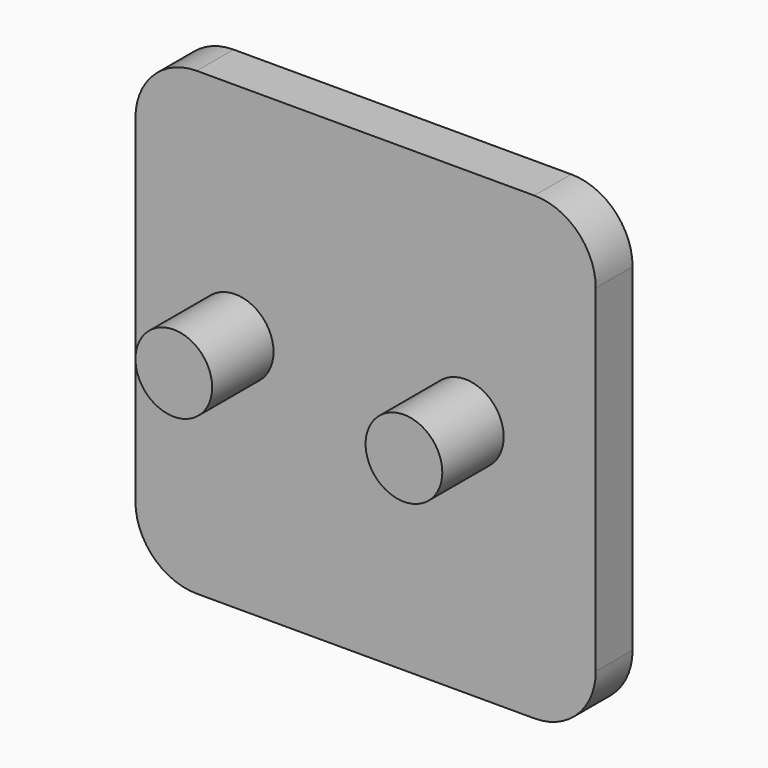
from build123d import *

# Parameters (mm, degrees)
F1_W           = 38.1
F1_H           = 38.1
F2_DEPTH       = 3.81
F3_R           = 3.175
F4_DEPTH       = 6.35
F5_R           = 5.08
F9_DEPTH       = 0.3175
F8_TEXT_SIZE   = 4.9309210024
F8_TEXT_SIZE_2 = 5.0353533071
F8_TEXT_SIZE_3 = 3.7948212897
F8_TEXT_SIZE_4 = 3.4233063666
F8_TEXT_SIZE_5 = 4.286538913
F8_TEXT_SIZE_6 = 3.7378385767
F8_TEXT_SIZE_7 = 4.2485771701
F8_TEXT_SIZE_8 = 4.0491771263
F10_DEPTH      = 0.3175
F11_W          = 23.3954964206
F11_H          = 0.4370380193
F12_DEPTH      = 0.3175


# Not quite as in the source:
# - Text() gives the source's letters only with a copy of the font that has no kerning and outlines rounded to 1/6400 em; it was checked with that copy


with BuildPart() as f2:
    # F1 (on offset) → F2 (new body)
    with BuildSketch(Plane.XZ.offset(25.4)):
        with Locations((-21.425308247, 18.5530144557)):
            Rectangle(F1_W, F1_H)
    extrude(amount=F2_DEPTH)

    # F3 (on face) → F4 (join)
    with BuildSketch(Plane.XZ.offset(29.21)):
        with Locations((-32.220308247, 19.1880144557)):
            Circle(F3_R)
        with Locations((-13.170308247, 19.1880144557)):
            Circle(F3_R)
    extrude(amount=F4_DEPTH)

    # F5
    f5_edges = [f2.edges().sort_by_distance(p)[0] for p in [
        (-40.475308, -27.305, 37.603014),
        (-2.375308, -27.305, 37.603014),
        (-40.475308, -27.305, -0.496986),
        (-2.375308, -27.305, -0.496986),
    ]]
    fillet(f5_edges, radius=F5_R)

    # F7 (on face) → F9 (cut)
    with BuildSketch(Plane(origin=(0, -25.4, 0), x_dir=(-1, 0, 0), z_dir=(0, 1, 0))):
        Polygon((12.6290200278, 34.7187258303), (3.9102202281, 34.7187258303), (6.485377904, 30.033910647), (6.8833935075, 5.9753647074), (6.922697669, 3.5995759973), (7.0077003911, 3.6009822506), (9.9715990946, 3.3956870902), (19.0850868821, 3.3956870902), (21.8502487987, 1.3529333519), (24.1223294288, 3.4225911368), (33.3103425801, 3.4225911368), (36.4377573133, 3.7207957357), (36.4377573133, 6.6668614745), (36.4377573133, 30.2996654063), (38.733985275, 34.526322037), (30.3983259946, 34.526322037), (30.0873341929, 34.526322037), (28.7930704653, 33.3972908556), (27.6523139328, 34.7049959274), (15.4967862216, 34.7049959274), (13.875534758, 33.2902558148), align=None)
    extrude(amount=-F9_DEPTH, mode=Mode.SUBTRACT)

    # F11 (on face) → F12 (join)
    with BuildSketch(Plane(origin=(0, -25.7175, 0), x_dir=(-1, 0, 0), z_dir=(0, 1, 0))):
        Polygon((33.4452651441, 31.8002551794), (9.1137969866, 31.8002551794), (9.1137969866, 31.0502536595), (33.4361046553, 31.0502536595), align=None)
        with Locations((21.4764908887, 25.272234343)):
            Rectangle(F11_W, F11_H)
        Polygon((33.1404767931, 6.2463656068), (17.2851830721, 24.3508461863), (16.5846580667, 23.7373500039), (32.3622695158, 5.7215714823), align=None)
        Polygon((25.6654638797, 4.1531343013), (11.0986828804, 21.7329673469), (10.5251273047, 21.2577149119), (24.9211379517, 3.8839750506), align=None)
    extrude(amount=F12_DEPTH)


with BuildPart() as f10:
    # F8 (on face) → F10 (new body)
    with BuildSketch(Plane(origin=(0, -25.4, 0), x_dir=(-1, 0, 0), z_dir=(0, 1, 0))):
        with Locations((8.5596432909, 26.6461465508)):
            Text('NEW YORK', F8_TEXT_SIZE, font='Open Sans', text_align=(TextAlign.LEFT, TextAlign.BOTTOM))
        with Locations((12.3642468825, 20.8774860948)):
            Text('R', F8_TEXT_SIZE_2, font='Open Sans', text_align=(TextAlign.LEFT, TextAlign.BOTTOM))
        with Locations((15.7174774754, 18.1452147663)):
            Text('A', F8_TEXT_SIZE_3, font='Open Sans', text_align=(TextAlign.LEFT, TextAlign.BOTTOM))
        with Locations((18.3649582658, 15.6804341823)):
            Text('N', F8_TEXT_SIZE_4, font='Open Sans', text_align=(TextAlign.LEFT, TextAlign.BOTTOM))
        with Locations((20.8318784163, 12.5941261649)):
            Text('G', F8_TEXT_SIZE_5, font='Open Sans', text_align=(TextAlign.LEFT, TextAlign.BOTTOM))
        with Locations((23.9168468902, 9.9028823897)):
            Text('E', F8_TEXT_SIZE_6, font='Open Sans', text_align=(TextAlign.LEFT, TextAlign.BOTTOM))
        with Locations((26.0135407168, 6.8439068273)):
            Text('R', F8_TEXT_SIZE_7, font='Open Sans', text_align=(TextAlign.LEFT, TextAlign.BOTTOM))
        with Locations((28.842827576, 3.9284992963)):
            Text('S', F8_TEXT_SIZE_8, font='Open Sans', text_align=(TextAlign.LEFT, TextAlign.BOTTOM))
    extrude(amount=F10_DEPTH)


solid = Compound([f2.part, f10.part])
